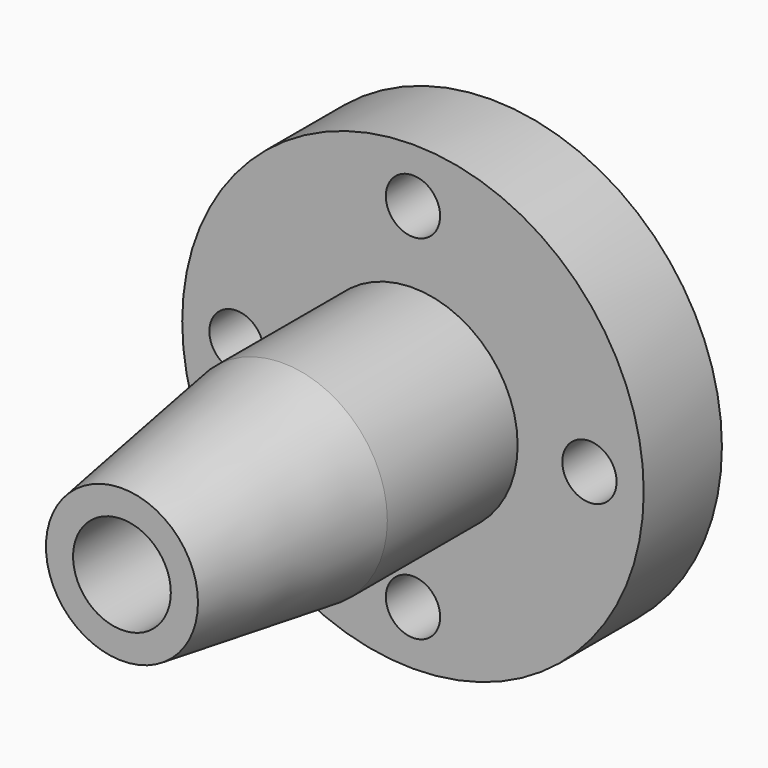
from build123d import *

# Parameters (mm, degrees)
F3_D            = 10
F3_COPIES_COUNT = 4


# Not quite as in the source:
# - a pattern or mirror of a feature is missing from the dataset's text; its kind, count and spacing are read off the source's solid


with BuildPart() as f1:
    # F0 (on Top) → F1 (revolve)
    with BuildSketch(Plane.XY):
        Polygon((42.5, 60.944458911), (9, 60.944458911), (9, -24.055541089), (14, -24.055541089), (19.277993122, 12.944458911), (19.277993122, 42.944458911), (42.5, 42.944458911), align=None)
    revolve(axis=Axis((0, 17.8779862242, 0), (0, -1, 0)))

    # F3 (through all)
    with Locations(Plane.XZ.offset(-42.944458911)):
        with Locations((32.5, 0)):
            f3 = Hole(F3_D / 2)

    # F3_copies: F3 ×4 about axis
    f3_copies_axis = Axis((0, 0, 0), (0, 1, 0))
    for i in range(1, F3_COPIES_COUNT):
        add(f3.rotate(f3_copies_axis, i * 360 / F3_COPIES_COUNT), mode=Mode.SUBTRACT)


solid = f1.part
